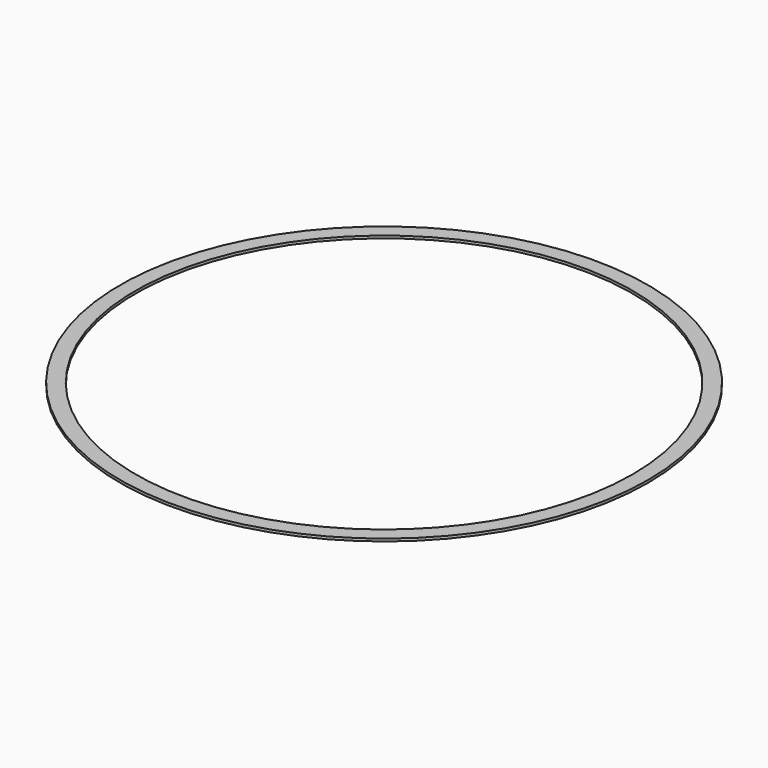
from build123d import *

# Parameters (mm, degrees)
F0_R     = 436.44566
F0_R_2   = 411.04566
F1_DEPTH = 4.2333333333


# Not quite as in the source:
# - a length typed as a fraction of an inch, garbled in the dataset ("3 / 203.2 mm" for 3/8 in), is restored


with BuildPart() as f1:
    # F0 (on Top) → F1 (new body)
    with BuildSketch(Plane.XY):
        Circle(F0_R)
        Circle(F0_R_2, mode=Mode.SUBTRACT)
    extrude(amount=F1_DEPTH)


solid = f1.part
